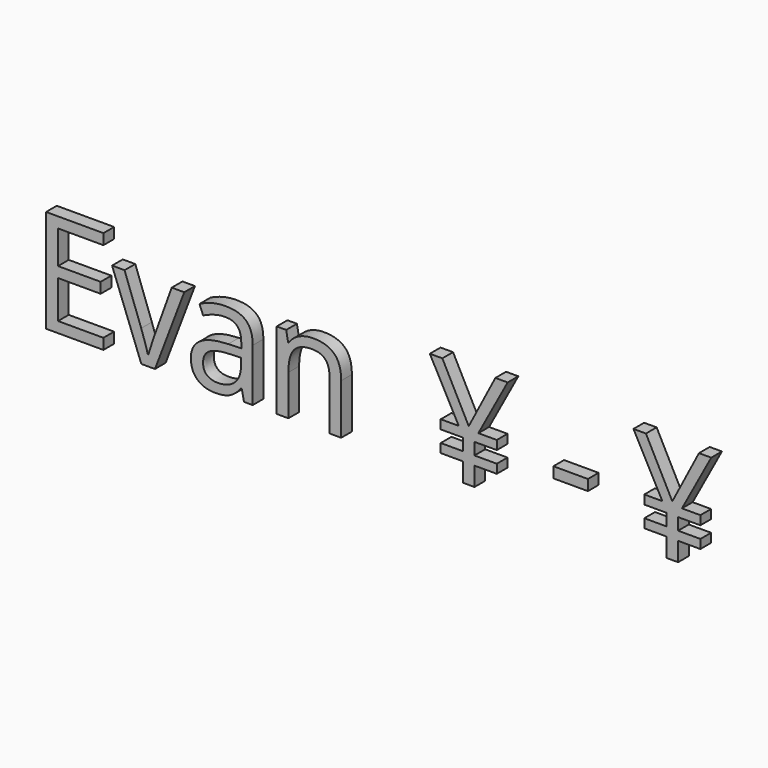
from build123d import *

# Parameters (mm, degrees)
F0_TEXT_SIZE = 820.3418304523
F1_DEPTH     = 76.2


# Not quite as in the source:
# - Text() gives the source's letters only with a copy of the font that has no kerning and outlines rounded to 1/6400 em; it was checked with that copy


with BuildPart() as f1:
    # F0 (on Front) → F1 (new body)
    with BuildSketch(Plane.XZ):
        with Locations((-692.433655262, -296.4707016945)):
            Text('Evan  ¥ - ¥', F0_TEXT_SIZE, font='Open Sans', text_align=(TextAlign.LEFT, TextAlign.BOTTOM))
    extrude(amount=F1_DEPTH)


solid = f1.part
